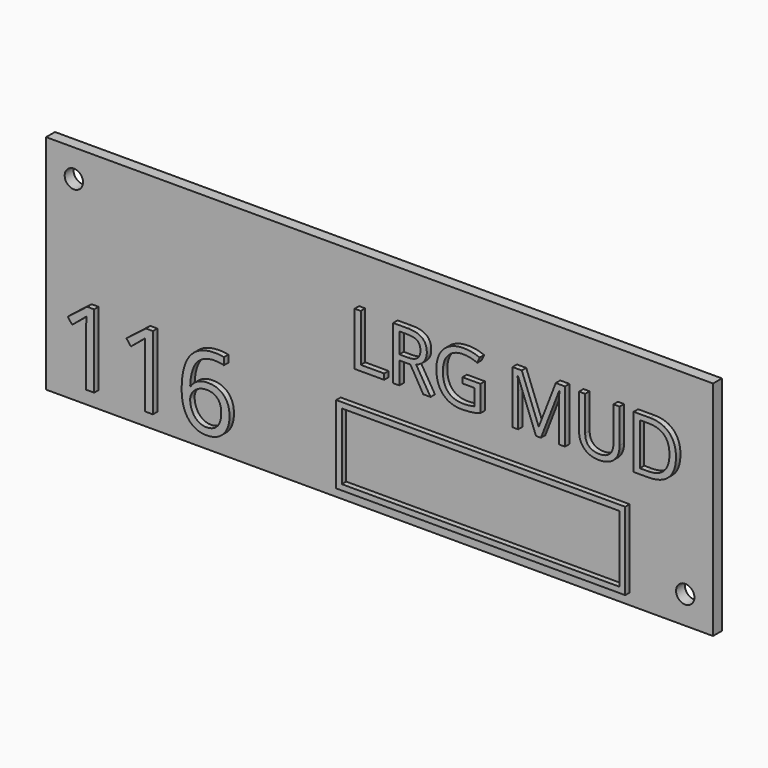
from build123d import *

# Parameters (mm, degrees)
F0_W         = 120
F0_H         = 40
F1_DEPTH     = 2
F3_D         = 3.3
F4_TEXT_SIZE = 13.3672155115
F5_DEPTH     = 1
F6_TEXT_SIZE = 18.4837545126
F7_DEPTH     = 1
F8_W         = 52
F8_H         = 14
F8_W_2       = 49.99999962
F8_H_2       = 11.99999962
F9_DEPTH     = 1


# Not quite as in the source:
# - Text() gives the source's letters only with a copy of the font that has no kerning and outlines rounded to 1/6400 em; it was checked with that copy


with BuildPart() as f1:
    # F0 (on Front) → F1 (new body)
    with BuildSketch(Plane.XZ):
        Rectangle(F0_W, F0_H)
    extrude(amount=F1_DEPTH)

    # F3 (through all)
    with Locations(Plane.XZ.offset(2)):
        with Locations((-55, 15), (55, -15)):
            Hole(F3_D / 2)

    # F4 (on face) → F5 (join)
    with BuildSketch(Plane.XZ.offset(2)):
        with Locations((-5, 2)):
            Text('LRG MUD', F4_TEXT_SIZE, font='Open Sans', text_align=(TextAlign.LEFT, TextAlign.BOTTOM))
    extrude(amount=F5_DEPTH)

    # F6 (on face) → F7 (join)
    with BuildSketch(Plane.XZ.offset(2)):
        with Locations((-57, -17)):
            Text('116', F6_TEXT_SIZE, font='Open Sans', text_align=(TextAlign.LEFT, TextAlign.BOTTOM))
    extrude(amount=F7_DEPTH)

    # F8 (on face) → F9 (join)
    with BuildSketch(Plane.XZ.offset(2)):
        with Locations((19, -11)):
            Rectangle(F8_W, F8_H)
        with Locations((19, -11)):
            Rectangle(F8_W_2, F8_H_2, mode=Mode.SUBTRACT)
    extrude(amount=F9_DEPTH)


solid = f1.part
